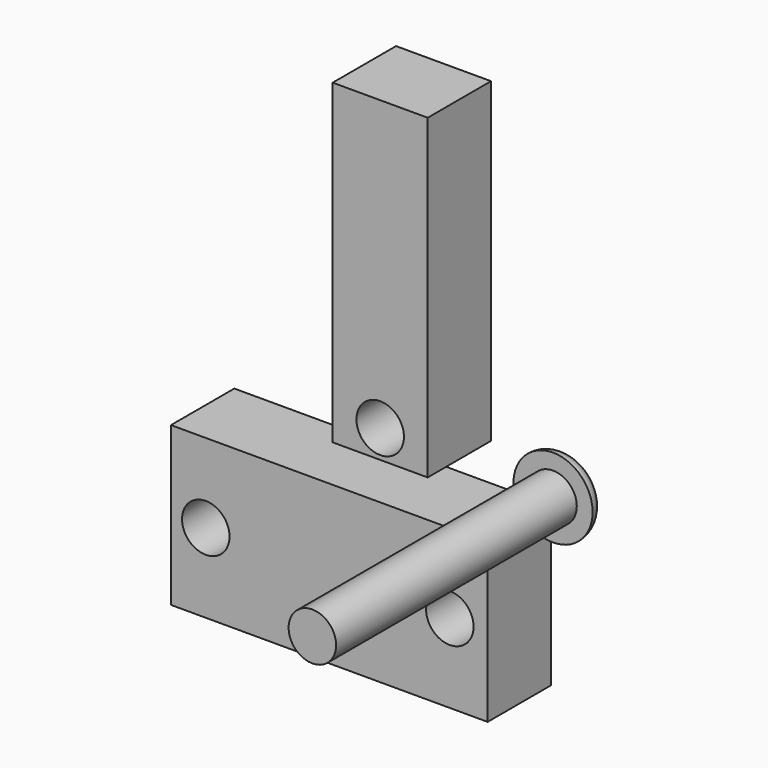
from build123d import *

# Parameters (mm, degrees)
F0_W     = 100
F0_H     = 50
F0_R     = 7.5
F1_DEPTH = 25
F2_W     = 30
F2_H     = 100
F2_R     = 7.5
F3_DEPTH = 25
F4_R     = 7.5
F5_DEPTH = 100
F6_R     = 12.5
F7_DEPTH = 5
F8_R     = 4.99999


# Not quite as in the source:
# - a fillet or chamfer is up to 0.001 mm smaller than in the source, because OpenCascade refuses the exact size


with BuildPart() as f1:
    # F0 (on Front) → F1 (new body)
    with BuildSketch(Plane.XZ):
        Rectangle(F0_W, F0_H)
        with Locations((-39.0076674521, 0)):
            Circle(F0_R, mode=Mode.SUBTRACT)
        with Locations((38.0539149046, 0)):
            Circle(F0_R, mode=Mode.SUBTRACT)
    extrude(amount=F1_DEPTH)


with BuildPart() as f3:
    # F2 (on Front) → F3 (new body)
    with BuildSketch(Plane.XZ):
        with Locations((16.0711699724, 86.8074811995)):
            Rectangle(F2_W, F2_H)
        with Locations((16.0711699724, 45.6409826875)):
            Circle(F2_R, mode=Mode.SUBTRACT)
    extrude(amount=F3_DEPTH)


with BuildPart() as f5:
    # F4 (on Front) → F5 (new body)
    with BuildSketch(Plane.XZ):
        with Locations((54.6516440809, 30.7668615133)):
            Circle(F4_R)
    extrude(amount=F5_DEPTH)

    # F6 (on Front) → F7 (join)
    with BuildSketch(Plane.XZ):
        with Locations((54.6516440809, 30.7668615133)):
            Circle(F6_R)
    extrude(amount=F7_DEPTH)

    # F8 (radius 5 in the source; OpenCascade refuses exactly that, so slightly less here)
    f8_edges = [f5.edges().sort_by_distance(p)[0] for p in [
        (42.151644, 0, 30.766862),
    ]]
    fillet(f8_edges, radius=F8_R)


solid = Compound([f1.part, f3.part, f5.part])
